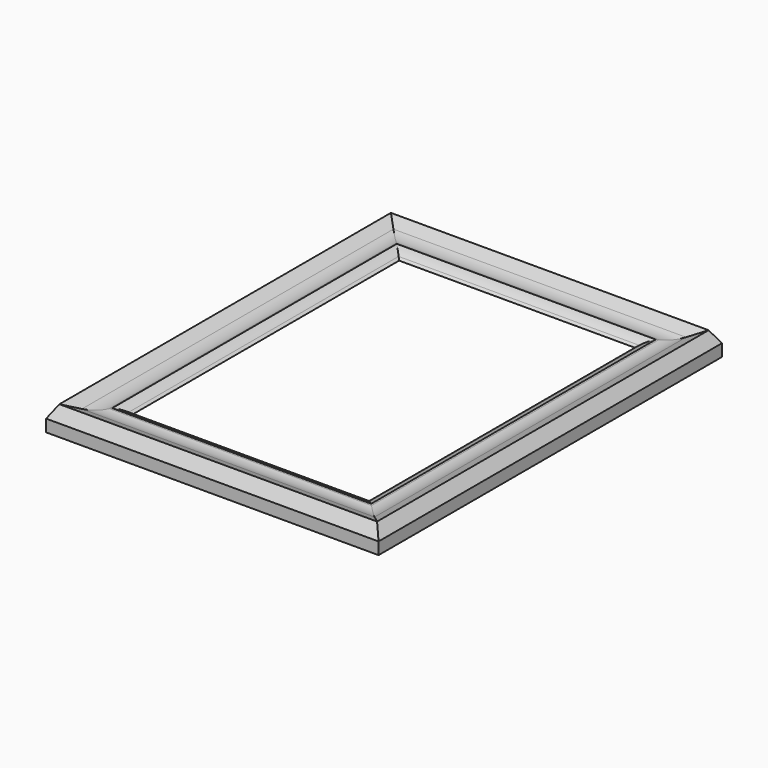
from build123d import *

# Parameters (mm, degrees)
F4_R     = 1.5875
F5_DEPTH = 0.79375


# Not quite as in the source:
# - a length typed as a fraction of an inch, garbled in the dataset ("3 / 203.2 mm" for 3/8 in), is restored


with BuildPart() as f2:
    # F2: sweep along a path in F0
    with BuildLine(Plane.XY) as f2_path:
        Line((35.71875, -48.41875), (35.71875, 48.41875))
        Line((35.71875, 48.41875), (-35.71875, 48.41875))
        Line((-35.71875, 48.41875), (-35.71875, -48.41875))
        Line((-35.71875, -48.41875), (35.71875, -48.41875))
    # F1 (on Front) → F2 (sweep)
    with BuildSketch(Plane.XZ):
        with BuildLine():
            Line((31.6033883161, 0.4986022927), (30.95625, 0))
            Line((30.95625, 0), (35.71875, 0))
            Line((35.71875, 0), (35.71875, -3.175))
            Line((35.71875, -3.175), (43.65625, -3.175))
            Line((43.65625, -3.175), (43.65625, 0))
            Line((43.65625, 0), (41.7148061097, 3.175))
            Line((41.7148061097, 3.175), (38.4218543283, 1.8180225684))
            ThreePointArc((38.4218543283, 1.8180225684), (36.4440586883, 1.3544374061), (34.4210724061, 1.5391352618))
            Line((34.4210724061, 1.5391352618), (34.0052636218, 1.6460575328))
            Line((34.0052636218, 1.6460575328), (33.899012953, 1.618762617))
            ThreePointArc((33.899012953, 1.618762617), (32.6942949799, 1.1753032814), (31.6033883161, 0.4986022927))
        make_face()
    sweep(path=f2_path.line, transition=Transition.RIGHT)

    # F4 (on face) → F5 (cut)
    with BuildSketch(Plane(origin=(0, 0, -3.175), x_dir=(1, 0, 0), z_dir=(0, 0, -1))):
        with Locations((-14.5520833333, 52.3875)):
            Circle(F4_R)
        with Locations((0, 52.3875)):
            Circle(F4_R)
        with Locations((14.5520833333, 52.3875)):
            Circle(F4_R)
        with Locations((-14.5520833333, -52.3875)):
            Circle(F4_R)
        with Locations((0, -52.3875)):
            Circle(F4_R)
        with Locations((14.5520833333, -52.3875)):
            Circle(F4_R)
    extrude(amount=-F5_DEPTH, mode=Mode.SUBTRACT)


solid = f2.part
